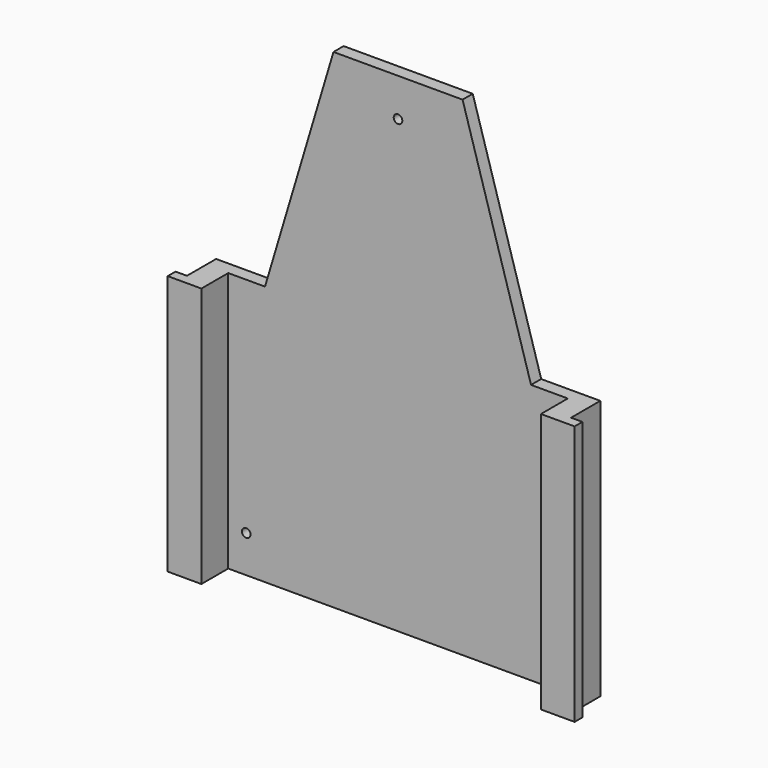
from build123d import *

# Parameters (mm, degrees)
F0_W     = 2.9037779868
F0_H     = 66.5
F1_DEPTH = 2.5
F2_DEPTH = 9.33
F3_R     = 1.1
F4_DEPTH = 3.25


# Not quite as in the source:
# - a feature names something its author has since deleted; it is built from what else it names


with BuildPart() as f1:
    # F0 (on Front) → F1 (new body)
    with BuildSketch(Plane.XZ):
        with Locations((-24.4931335896, -18.415993683)):
            Rectangle(F0_W, F0_H)
        Polygon((-20.845022583, 14.834006317), (-23.0412445962, 14.834006317), (-23.0412445962, -51.665993683), (-17.345022583, -51.665993683), (-17.345022583, 14.834006317), align=None)
    extrude(amount=F1_DEPTH)

    # F0 (on Front) → F2, piece 2 (join)
    with BuildSketch(Plane.XZ):
        Polygon((-20.845022583, 14.834006317), (-23.0412445962, 14.834006317), (-23.0412445962, -51.665993683), (-17.345022583, -51.665993683), (-17.345022583, 14.834006317), align=None)
    extrude(amount=-F2_DEPTH)



with BuildPart() as f1b:
    # F0 (on Front) → F1, piece 2 (new body)
    with BuildSketch(Plane.XZ):
        with Locations((76.6030884236, -18.415993683)):
            Rectangle(F0_W, F0_H)
        Polygon((72.954977417, 14.834006317), (69.454977417, 14.834006317), (69.454977417, -51.665993683), (75.1511994302, -51.665993683), (75.1511994302, 14.834006317), align=None)
    extrude(amount=F1_DEPTH)

    # F0 (on Front) → F2 (join)
    with BuildSketch(Plane.XZ):
        Polygon((72.954977417, 14.834006317), (69.454977417, 14.834006317), (69.454977417, -51.665993683), (75.1511994302, -51.665993683), (75.1511994302, 14.834006317), align=None)
    extrude(amount=-F2_DEPTH)


with BuildPart() as f1_1:
    add(f1.part)

    add(f1b.part)  # F4 merges F1b
    # F3 (on face) → F4 (join)
    with BuildSketch(Plane(origin=(0, 9.33, 0), x_dir=(-1, 0, 0), z_dir=(0, 1, 0))):
        Polygon((17.345022583, -51.665993683), (17.345022583, 14.834006317), (7.945022583, 14.834006317), (-26.054977417, 14.834006317), (-60.054977417, 14.834006317), (-75.1511994302, 14.834006317), (-75.1511994302, -51.665993683), align=None)
        with Locations((-64.854977417, -42.165993683)):
            Circle(F3_R, mode=Mode.SUBTRACT)
        with Locations((12.745022583, -42.165993683)):
            Circle(F3_R, mode=Mode.SUBTRACT)
        Polygon((-26.054977417, 14.834006317), (7.945022583, 14.834006317), (-9.554977417, 73.334006317), (-26.054977417, 73.334006317), (-42.554977417, 73.334006317), (-60.054977417, 14.834006317), align=None)
        with Locations((-26.054977417, 63.584006317)):
            Circle(F3_R, mode=Mode.SUBTRACT)
    extrude(amount=-F4_DEPTH)


solid = f1_1.part
